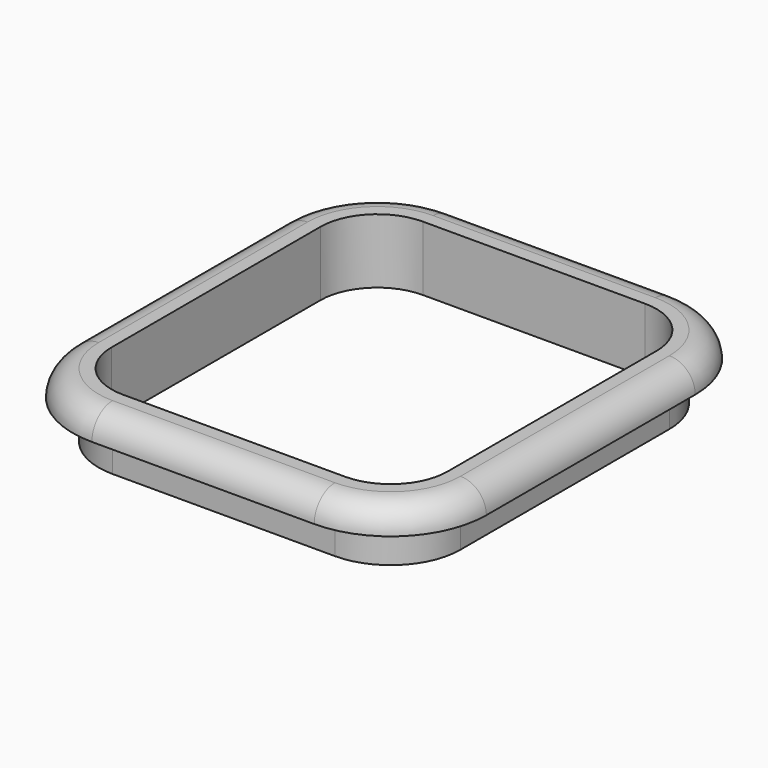
from build123d import *

# Parameters (mm, degrees)
F1_DEPTH = 15
F2_DEPTH = 10
F3_R     = 9.99999


# Not quite as in the source:
# - a fillet or chamfer is up to 0.001 mm smaller than in the source, because OpenCascade refuses the exact size
# - a feature of the source that left no trace in its solid (it failed there, or was rolled back) is left out


with BuildPart() as f1:
    # F0 (on Top) → F1 (new body)
    with BuildSketch(Plane.XY):
        with BuildLine():
            Line((-43, -77.5), (43, -77.5))
            ThreePointArc((43, -77.5), (62.091883092, -69.591883092), (70, -50.5))
            Line((70, -50.5), (70, 50.5))
            ThreePointArc((70, 50.5), (62.091883092, 69.591883092), (43, 77.5))
            Line((43, 77.5), (-43, 77.5))
            ThreePointArc((-43, 77.5), (-62.091883092, 69.591883092), (-70, 50.5))
            Line((-70, 50.5), (-70, -50.5))
            ThreePointArc((-70, -50.5), (-62.091883092, -69.591883092), (-43, -77.5))
        make_face()
        with BuildLine():
            Line((64.9999988648, 50.5), (64.9999988648, -50.5))
            ThreePointArc((64.9999988648, -50.5), (58.5563483834, -66.0563483834), (43, -72.4999988648))
            Line((43, -72.4999988648), (-43, -72.4999988648))
            ThreePointArc((-43, -72.4999988648), (-58.5563483834, -66.0563483834), (-64.9999988648, -50.5))
            Line((-64.9999988648, -50.5), (-64.9999988648, 50.5))
            ThreePointArc((-64.9999988648, 50.5), (-58.5563483834, 66.0563483834), (-43, 72.4999988648))
            Line((-43, 72.4999988648), (43, 72.4999988648))
            ThreePointArc((43, 72.4999988648), (58.5563483834, 66.0563483834), (64.9999988648, 50.5))
        make_face(mode=Mode.SUBTRACT)
    extrude(amount=-F1_DEPTH)

    # F0 (on Top) → F2 (join)
    with BuildSketch(Plane.XY):
        with BuildLine():
            Line((80, -50.5), (80, 50.5))
            ThreePointArc((80, 50.5), (69.1629509039, 76.6629509039), (43, 87.5))
            Line((43, 87.5), (-43, 87.5))
            ThreePointArc((-43, 87.5), (-69.1629509039, 76.6629509039), (-80, 50.5))
            Line((-80, 50.5), (-80, -50.5))
            ThreePointArc((-80, -50.5), (-69.1629509039, -76.6629509039), (-43, -87.5))
            Line((-43, -87.5), (43, -87.5))
            ThreePointArc((43, -87.5), (69.1629509039, -76.6629509039), (80, -50.5))
        make_face()
        with BuildLine():
            ThreePointArc((70, -50.5), (62.091883092, -69.591883092), (43, -77.5))
            Line((43, -77.5), (-43, -77.5))
            ThreePointArc((-43, -77.5), (-62.091883092, -69.591883092), (-70, -50.5))
            Line((-70, -50.5), (-70, 50.5))
            ThreePointArc((-70, 50.5), (-62.091883092, 69.591883092), (-43, 77.5))
            Line((-43, 77.5), (43, 77.5))
            ThreePointArc((43, 77.5), (62.091883092, 69.591883092), (70, 50.5))
            Line((70, 50.5), (70, -50.5))
        make_face(mode=Mode.SUBTRACT)
        with BuildLine():
            Line((-43, -77.5), (43, -77.5))
            ThreePointArc((43, -77.5), (62.091883092, -69.591883092), (70, -50.5))
            Line((70, -50.5), (70, 50.5))
            ThreePointArc((70, 50.5), (62.091883092, 69.591883092), (43, 77.5))
            Line((43, 77.5), (-43, 77.5))
            ThreePointArc((-43, 77.5), (-62.091883092, 69.591883092), (-70, 50.5))
            Line((-70, 50.5), (-70, -50.5))
            ThreePointArc((-70, -50.5), (-62.091883092, -69.591883092), (-43, -77.5))
        make_face()
        with BuildLine():
            Line((64.9999988648, 50.5), (64.9999988648, -50.5))
            ThreePointArc((64.9999988648, -50.5), (58.5563483834, -66.0563483834), (43, -72.4999988648))
            Line((43, -72.4999988648), (-43, -72.4999988648))
            ThreePointArc((-43, -72.4999988648), (-58.5563483834, -66.0563483834), (-64.9999988648, -50.5))
            Line((-64.9999988648, -50.5), (-64.9999988648, 50.5))
            ThreePointArc((-64.9999988648, 50.5), (-58.5563483834, 66.0563483834), (-43, 72.4999988648))
            Line((-43, 72.4999988648), (43, 72.4999988648))
            ThreePointArc((43, 72.4999988648), (58.5563483834, 66.0563483834), (64.9999988648, 50.5))
        make_face(mode=Mode.SUBTRACT)
    extrude(amount=F2_DEPTH)

    # F3 (radius 10 in the source; OpenCascade refuses exactly that, so slightly less here)
    f3_edges = [f1.edges().sort_by_distance(p)[0] for p in [
        (-69.162951, -76.662951, 10),
        (80, 0, 10),
        (69.162951, 76.662951, 10),
        (0, 87.5, 10),
        (-69.162951, 76.662951, 10),
        (-80, 0, 10),
        (0, -87.5, 10),
        (69.162951, -76.662951, 10),
    ]]
    fillet(f3_edges, radius=F3_R)


solid = f1.part
